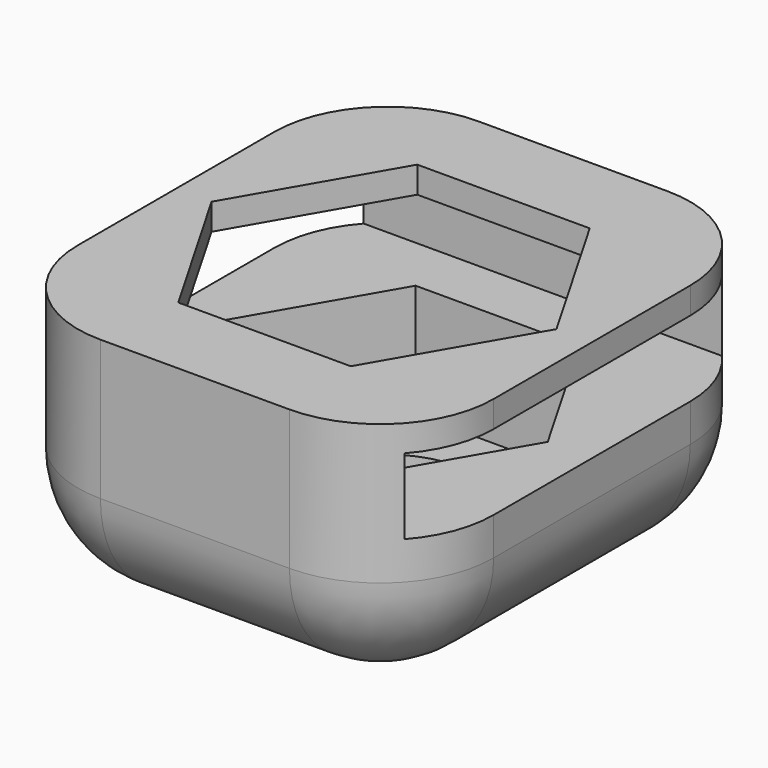
from build123d import *

# Parameters (mm, degrees)
F0_W        = 11
F0_H        = 12.5
F0_R        = 2.5
F1_DEPTH    = 4
F2_R        = 2.5
F3_DEPTH    = 3
F4_W        = 11
F4_H        = 1
F5_DEPTH    = 2
F6_W        = 11
F6_H        = 12.5
F7_DEPTH    = 0.7
F8_DEPTH    = 25
F9_T1_DEPTH = 21.7
F11_DEPTH   = 2
F12_R       = 2.99999


# Not quite as in the source:
# - a fillet or chamfer that OpenCascade refuses, or shapes differently, is made with other operations: its cross-section is extruded or revolved along the edge and cut away or added
# - a fillet or chamfer is up to 0.001 mm smaller than in the source, because OpenCascade refuses the exact size


with BuildPart() as f1:
    # F0 (on Top) → F1 (new body)
    with BuildSketch(Plane.XY):
        Rectangle(F0_W, F0_H)
        Circle(F0_R, mode=Mode.SUBTRACT)
    extrude(amount=-F1_DEPTH)

    # F2 (on Top) → F3 (cut)
    with BuildSketch(Plane.XY):
        Polygon((2.1650635095, 3.75), (-2.1650635095, 3.75), (-4.3301270189, 0), (-2.1650635095, -3.75), (2.1650635095, -3.75), (4.3301270189, 0), align=None)
        Circle(F2_R, mode=Mode.SUBTRACT)
    extrude(amount=-F3_DEPTH, mode=Mode.SUBTRACT)

    # F4 (on face) → F5 (join)
    with BuildSketch(Plane.XY):
        with Locations((0, 5.75)):
            Rectangle(F4_W, F4_H)
        with Locations((0, -5.75)):
            Rectangle(F4_W, F4_H)
    extrude(amount=F5_DEPTH)

    # F6 (on face) → F7 (join)
    with BuildSketch(Plane.XY.offset(2)):
        Rectangle(F6_W, F6_H)
    extrude(amount=F7_DEPTH)

    # F2 (on Top) → F8 (cut)
    with BuildSketch(Plane.XY):
        Polygon((2.1650635095, 3.75), (-2.1650635095, 3.75), (-4.3301270189, 0), (-2.1650635095, -3.75), (2.1650635095, -3.75), (4.3301270189, 0), align=None)
        Circle(F2_R, mode=Mode.SUBTRACT)
        Circle(F2_R)
    extrude(amount=F8_DEPTH, mode=Mode.SUBTRACT)

    # F9: fillet of radius 3 on 4 edges, made by hand

    # F9_s2 → F9_t1 (cut)
    with BuildSketch(Plane.XY.offset(-11.5)):
        with BuildLine():
            ThreePointArc((-2.5, -6.25), (-4.6213203436, -5.3713203436), (-5.5, -3.25))
            Line((-5.5, -3.25), (-5.5, -6.25))
            Line((-5.5, -6.25), (-2.5, -6.25))
        make_face()
        with BuildLine():
            ThreePointArc((2.5, -6.25), (4.6213203436, -5.3713203436), (5.5, -3.25))
            Line((5.5, -3.25), (5.5, -6.25))
            Line((5.5, -6.25), (2.5, -6.25))
        make_face()
        with BuildLine():
            ThreePointArc((5.5, 3.25), (4.6213203436, 5.3713203436), (2.5, 6.25))
            Line((2.5, 6.25), (5.5, 6.25))
            Line((5.5, 6.25), (5.5, 3.25))
        make_face()
        with BuildLine():
            ThreePointArc((-5.5, 3.25), (-4.6213203436, 5.3713203436), (-2.5, 6.25))
            Line((-2.5, 6.25), (-5.5, 6.25))
            Line((-5.5, 6.25), (-5.5, 3.25))
        make_face()
    extrude(amount=F9_T1_DEPTH, mode=Mode.SUBTRACT)

    # F10 (on face) → F11 (cut)
    with BuildSketch(Plane.XY.offset(2.7)):
        Polygon((2.2805335633, 3.95), (-2.2805335633, 3.95), (-4.5610671266, 0), (-2.2805335633, -3.95), (2.2805335633, -3.95), (4.5610671266, 0), align=None)
    extrude(amount=-F11_DEPTH, mode=Mode.SUBTRACT)

    # F12 (radius 3 in the source; OpenCascade refuses exactly that, so slightly less here)
    f12_edges = [f1.edges().sort_by_distance(p)[0] for p in [
        (0, -6.25, -4),
    ]]
    fillet(f12_edges, radius=F12_R)


solid = f1.part
